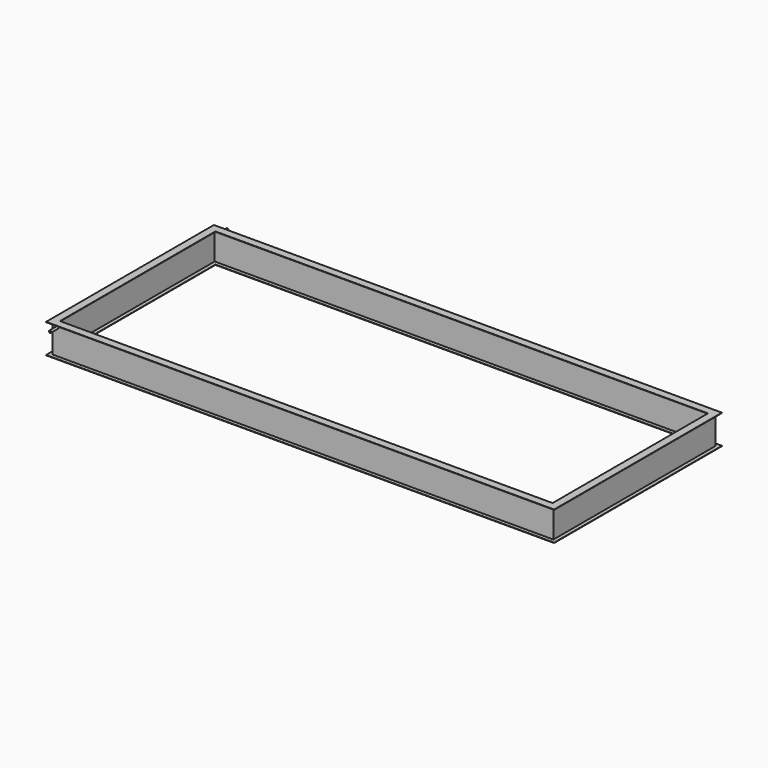
from build123d import *

# Parameters (mm, degrees)
F3_R     = 9.525
F4_DEPTH = 82.55
F5_R     = 9.525
F6_DEPTH = 82.55


with BuildPart() as f2:
    # F2: sweep along a path in F0
    with BuildLine(Plane.XY) as f2_path:
        Line((0, 0), (4368.8, 0))
        Line((4368.8, 0), (4368.8, 1803.4))
        Line((4368.8, 1803.4), (0, 1803.4))
        Line((0, 1803.4), (0, 0))
    # F1 (on Right) → F2 (sweep)
    with BuildSketch(Plane.YZ):
        Polygon((66.675, 0), (0, 0), (0, -3.175), (31.75, -3.175), (31.75, -250.825), (0, -250.825), (0, -254), (66.675, -254), (66.675, -250.825), (34.925, -250.825), (34.925, -3.175), (66.675, -3.175), align=None)
    sweep(path=f2_path.line, transition=Transition.RIGHT)

    # F3 (on face) → F4 (join)
    with BuildSketch(Plane.XZ.offset(-31.75)):
        with Locations((75, -30)):
            Circle(F3_R)
    extrude(amount=F4_DEPTH)

    # F5 (on face) → F6 (join)
    with BuildSketch(Plane(origin=(0, 1771.65, 0), x_dir=(-1, 0, 0), z_dir=(0, 1, 0))):
        with Locations((-75, -30)):
            Circle(F5_R)
    extrude(amount=F6_DEPTH)


solid = f2.part
